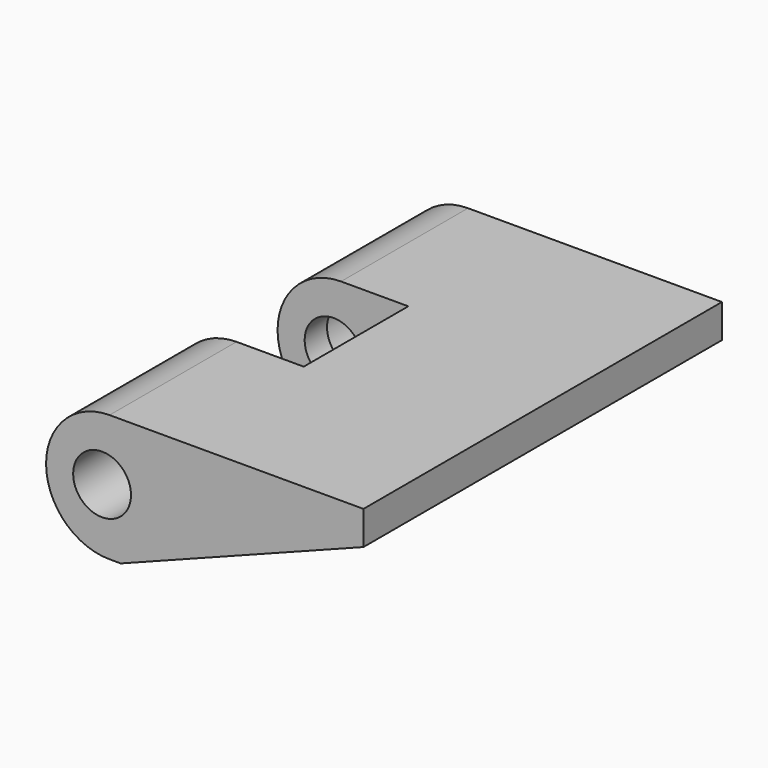
from build123d import *

# Parameters (mm, degrees)
F1_DEPTH    = 6.8
F2_R        = 3.39999
F3_R        = 1.55
F4_DEPTH    = 24.001
F3_R_2      = 2.05
F5_DEPTH    = 7
F0_W        = 8
F0_H        = 24
F6_DEPTH    = 6.8
F7_T1_DEPTH = 7
F8_T1_DEPTH = 91.4331581264


# Not quite as in the source:
# - a fillet or chamfer that OpenCascade refuses, or shapes differently, is made with other operations: its cross-section is extruded or revolved along the edge and cut away or added
# - a fillet or chamfer is up to 0.001 mm smaller than in the source, because OpenCascade refuses the exact size
# - a feature names something its author has since deleted; it is built from what else it names


with BuildPart() as f1:
    # F0 (on Top) → F1 (new body)
    with BuildSketch(Plane.XY):
        Polygon((-2, -12), (0, -12), (0, 12), (-2, 12), (-9, 12), (-9, 3.5), (-2, 3.5), (-2, -3.5), (-9, -3.5), (-9, -12), align=None)
    extrude(amount=F1_DEPTH)

    # F2 (radius 3.4 in the source; OpenCascade refuses exactly that, so slightly less here)
    f2_edges = [f1.edges().sort_by_distance(p)[0] for p in [
        (-9, 7.75, 6.8),
        (-9, 7.75, 0),
        (-9, -7.75, 0),
        (-9, -7.75, 6.8),
    ]]
    fillet(f2_edges, radius=F2_R)

    # F3 (on face) → F4 (cut, through all)
    with BuildSketch(Plane(origin=(0, 12, 0), x_dir=(-1, 0, 0), z_dir=(0, 1, 0))):
        with Locations((6, 3.4)):
            Circle(F3_R)
    extrude(amount=-F4_DEPTH, mode=Mode.SUBTRACT)

    # F3 (on face) → F5 (cut)
    with BuildSketch(Plane(origin=(0, 12, 0), x_dir=(-1, 0, 0), z_dir=(0, 1, 0))):
        with Locations((6, 3.4)):
            Circle(F3_R_2)
        with Locations((6, 3.4)):
            Circle(F3_R, mode=Mode.SUBTRACT)
    extrude(amount=-F5_DEPTH, mode=Mode.SUBTRACT)

    # F0 (on Top) → F6 (join, through all)
    with BuildSketch(Plane.XY):
        with Locations((4, 0)):
            Rectangle(F0_W, F0_H)
    extrude(amount=F6_DEPTH)

    # F7: fillet of radius 7 on 1 edges, made by hand

    # F7_s2 → F7_t1 (cut)
    with BuildSketch(Plane.XZ.offset(-3.5)):
        with BuildLine():
            ThreePointArc((-2.0003998352, 6.7999885178), (0.1189410708, 1.9796991069), (4.9980806884, -0.0004))
            Line((4.9980806884, -0.0004), (4.9980806884, -0.7005365685))
            ThreePointArc((4.9980806884, -0.7005365685), (1.4990403442, -0.7001365685), (-2, -0.7001365685))
            Line((-2, -0.7001365685), (-2.7001365685, 0))
            ThreePointArc((-2.7001365685, 0), (-2.7001365685, 3.3999942589), (-2.7002478875, 6.7798908011))
            Line((-2.7002478875, 6.7798908011), (-2.0003998352, 6.7999885178))
        make_face()
    extrude(amount=F7_T1_DEPTH, mode=Mode.SUBTRACT)

    # F8: chamfer of 5 x 13 on 1 edges, made by hand

    # F8_s2 → F8_t1 (cut)
    with BuildSketch(Plane.XZ.offset(-45.7165790632)):
        Polygon((8, 5), (-5, 0), (8, 0), align=None)
    extrude(amount=F8_T1_DEPTH, mode=Mode.SUBTRACT)


solid = f1.part
